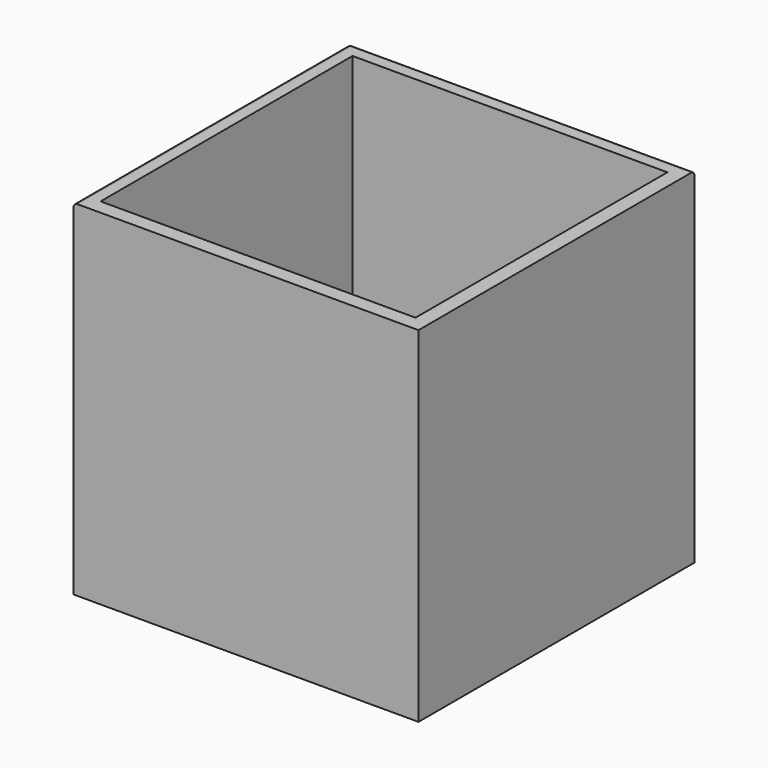
from build123d import *

# Parameters (mm, degrees)
F2_W     = 460
F2_H     = 460
F2_W_2   = 420
F2_H_2   = 420
F3_DEPTH = 460
F4_R     = 5
F5_R     = 5


# Not quite as in the source:
# - the program builds the solid bodies; features that only make, move or delete a surface that nothing else refers to are left out


with BuildPart() as f3:
    # F2 (on Top) → F3 (new body)
    with BuildSketch(Plane.XY):
        Rectangle(F2_W, F2_H)
        Rectangle(F2_W_2, F2_H_2, mode=Mode.SUBTRACT)
    extrude(amount=F3_DEPTH)

    # F4
    f4_edges = [f3.edges().sort_by_distance(p)[0] for p in [
        (-230, 230, 230),
    ]]
    fillet(f4_edges, radius=F4_R)

    # F5
    f5_edges = [f3.edges().sort_by_distance(p)[0] for p in [
        (-230, -2.5, 460),
    ]]
    fillet(f5_edges, radius=F5_R)


solid = f3.part
